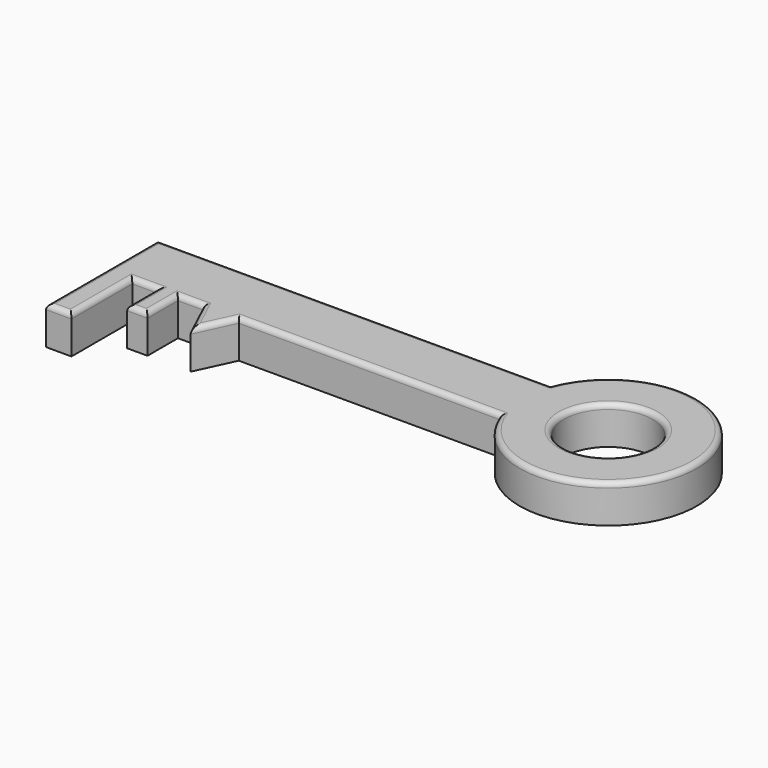
from build123d import *

# Parameters (mm, degrees)
F0_W     = 155
F0_H     = 12.5
F0_W_2   = 8
F0_H_2   = 15
F0_W_3   = 10
F0_H_3   = 30
F1_DEPTH = 15
F2_R     = 2


with BuildPart() as f1:
    # F0 (on Top) → F1 (new body)
    with BuildSketch(Plane.XY):
        with Locations((-59.8887689211, 33.75)):
            Rectangle(F0_W, F0_H)
        Polygon((17.6112310789, 27.5), (-137.3887689211, 27.5), (-137.3887689211, 15), (-127.3887689211, 15), (-117.3887689211, 15), (-109.3887689211, 15), (-99.3887689211, 15), (-85.3887689211, 15), (17.6112310789, 15), align=None)
        with BuildLine():
            ThreePointArc((17.6112310789, 15), (85.3029731554, 27.5), (17.6112310789, 40))
            Line((17.6112310789, 40), (17.6112310789, 27.5))
            Line((17.6112310789, 27.5), (17.6112310789, 15))
        make_face()
        with BuildLine():
            ThreePointArc((67.8029731554, 27.5), (50.3029731554, 10), (32.8029731554, 27.5))
            ThreePointArc((32.8029731554, 27.5), (50.3029731554, 45), (67.8029731554, 27.5))
        make_face(mode=Mode.SUBTRACT)
        Polygon((-92.3888981342, 0), (-85.3887689211, 15), (-99.3887689211, 15), align=None)
        with Locations((-113.3887689211, 7.5)):
            Rectangle(F0_W_2, F0_H_2)
        with Locations((-132.3887689211, 0)):
            Rectangle(F0_W_3, F0_H_3)
    extrude(amount=F1_DEPTH)

    # F2
    f2_edges = [f1.edges().sort_by_distance(p)[0] for p in [
        (-59.888769, 40, 15),
        (85.302973, 27.5, 15),
        (-33.888769, 15, 15),
        (-88.888834, 7.5, 15),
        (-122.388769, 15, 15),
        (-109.388769, 7.5, 15),
        (-132.388769, -15, 15),
        (-127.388769, 0, 15),
        (-137.388769, 12.5, 15),
        (-113.388769, 0, 15),
        (-117.388769, 7.5, 15),
        (-95.888834, 7.5, 15),
        (67.802973, 27.5, 15),
        (-104.388769, 15, 15),
    ]]
    fillet(f2_edges, radius=F2_R)


solid = f1.part
